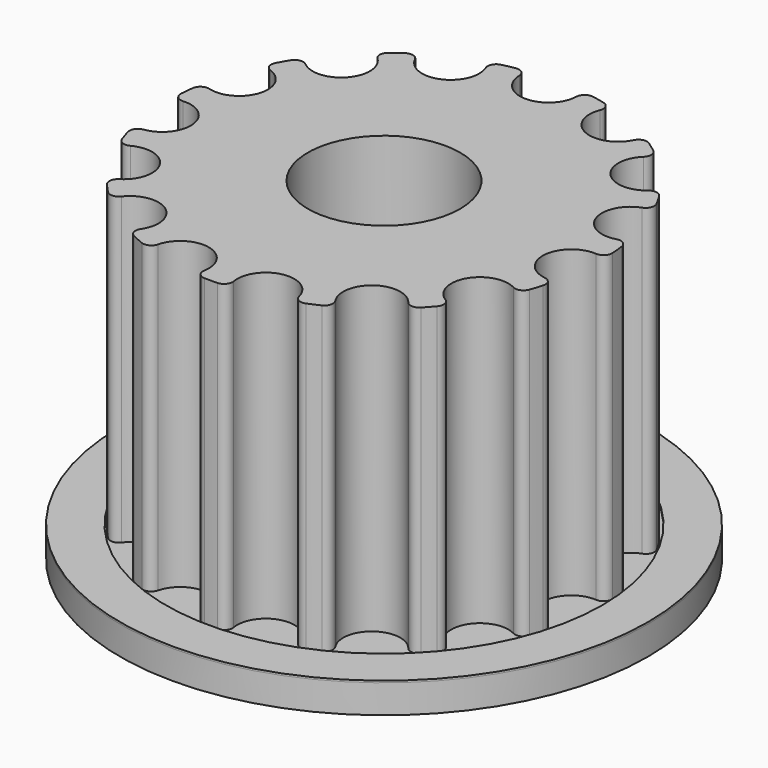
from build123d import *

# Parameters (mm, degrees)
F2_R            = 11.3641207455
F3_DEPTH        = 16
F5_DEPTH        = 16
F5_COPIES_COUNT = 15
F8_R            = 13.8641207455
F8_R_2          = 11.3641207455
F9_DEPTH        = 1.5
F7_R            = 4
F10_DEPTH       = 17.501
F11_R           = 13.8641207455
F11_R_2         = 11.4641207455
F12_DEPTH       = 0.1


# Not quite as in the source:
# - a feature of the source that left no trace in its solid (it failed there, or was rolled back) is left out
# - a pattern or mirror of a feature is missing from the dataset's text; its kind, count and spacing are read off the source's solid


with BuildPart() as f3:
    # F2 (on Top) → F3 (new body)
    with BuildSketch(Plane.XY):
        Circle(F2_R)
    extrude(amount=F3_DEPTH)

    # F4 (on face) → F5 (cut, through all)
    with BuildSketch(Plane.XY.offset(16)):
        with BuildLine():
            ThreePointArc((-2.0292576741, 11.181473678), (-1.6663457301, 11.0889370809), (-1.4991557657, 10.7538018594))
            ThreePointArc((-1.4991557657, 10.7538018594), (0, 9.3041207455), (1.4991557657, 10.7538018594))
            ThreePointArc((1.4991557657, 10.7538018594), (1.6663457301, 11.0889370809), (2.0292576741, 11.181473678))
            ThreePointArc((2.0292576741, 11.181473678), (0, 11.3641207455), (-2.0292576741, 11.181473678))
        make_face()
    f5 = extrude(amount=-F5_DEPTH, mode=Mode.SUBTRACT)

    # F5_copies: F5 ×15 about axis
    f5_copies_axis = Axis((0, 0, 0), (0, 0, 1))
    for i in range(1, F5_COPIES_COUNT):
        add(f5.rotate(f5_copies_axis, i * 360 / F5_COPIES_COUNT), mode=Mode.SUBTRACT)

    # F8 (on face) + F2 (on Top) → F9 (join)
    with BuildSketch(Plane.XY):
        Circle(F8_R)
        Circle(F8_R_2, mode=Mode.SUBTRACT)
    with BuildSketch(Plane.XY):
        Circle(F2_R)
    extrude(amount=-F9_DEPTH)

    # F7 (on face) → F10 (cut, through all)
    with BuildSketch(Plane.XY.offset(16)):
        Circle(F7_R)
    extrude(amount=-F10_DEPTH, mode=Mode.SUBTRACT)

    # F11 (on face) → F12 (join)
    with BuildSketch(Plane.XY):
        Circle(F11_R)
        Circle(F11_R_2, mode=Mode.SUBTRACT)
    extrude(amount=F12_DEPTH)


solid = f3.part
